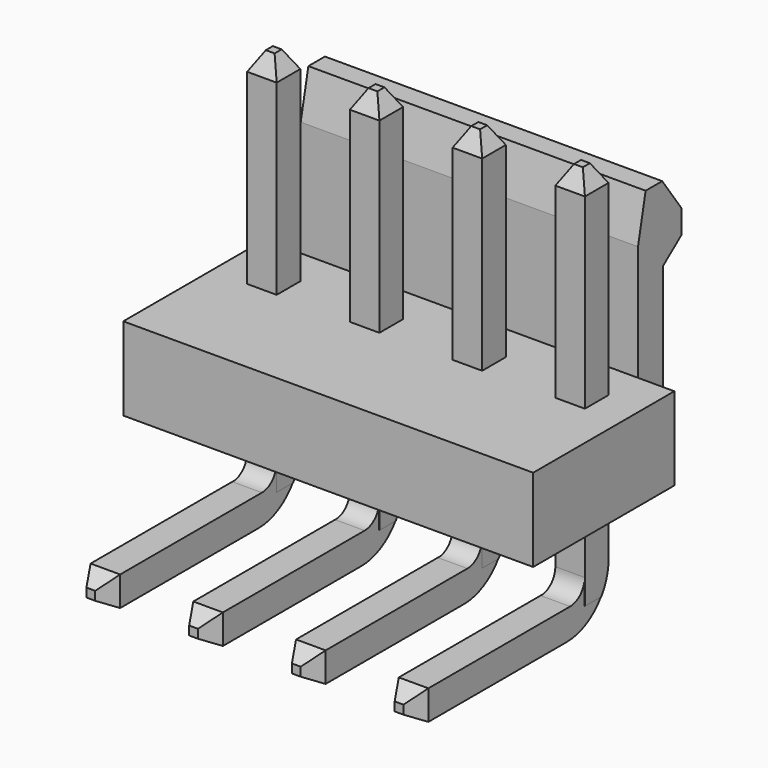
from build123d import *

# Parameters (mm, degrees)
F0_W          = 6.8
F0_H          = 3.2
F1_DEPTH      = 7.9
F1_DEPTH_BACK = 7.9
F2_DEPTH      = 6.5
F2_DEPTH_BACK = 6.5
F3_W          = 1.14
F3_H          = 1.14
F4_DEPTH      = 11.1
F4_DEPTH_BACK = 3.5
F5_C1_SIZE2   = 0.4
F5_C1_SIZE    = 0.7
F5_C2_SIZE2   = 0.7
F5_C2_SIZE    = 0.4
F5_C3_SIZE2   = 0.7
F5_C3_SIZE    = 0.4
F5_C4_SIZE2   = 0.7
F5_C4_SIZE    = 0.4
F5_2_C1_SIZE2 = 0.4
F5_2_C1_SIZE  = 0.7
F5_2_C2_SIZE2 = 0.7
F5_2_C2_SIZE  = 0.4
F5_2_C3_SIZE2 = 0.7
F5_2_C3_SIZE  = 0.4
F5_2_C4_SIZE2 = 0.7
F5_2_C4_SIZE  = 0.4
F5_3_C1_SIZE2 = 0.4
F5_3_C1_SIZE  = 0.7
F5_3_C2_SIZE2 = 0.7
F5_3_C2_SIZE  = 0.4
F5_3_C3_SIZE2 = 0.7
F5_3_C3_SIZE  = 0.4
F5_3_C4_SIZE2 = 0.7
F5_3_C4_SIZE  = 0.4
F5_4_C1_SIZE2 = 0.4
F5_4_C1_SIZE  = 0.7
F5_4_C2_SIZE2 = 0.7
F5_4_C2_SIZE  = 0.4
F5_4_C3_SIZE2 = 0.7
F5_4_C3_SIZE  = 0.4
F5_4_C4_SIZE2 = 0.7
F5_4_C4_SIZE  = 0.4
F6_W          = 1.14
F6_H          = 1.14
F7_DEPTH      = 8.8
F7_DEPTH_BACK = 0.57
F8_R          = 0.7
F8_2_R        = 0.7
F8_3_R        = 0.7
F8_4_R        = 0.7
F9_T1_DEPTH   = 11.14
F9_2_T1_DEPTH = 11.14
F9_3_T1_DEPTH = 11.14
F9_4_T1_DEPTH = 11.14
F10_SIZE2     = 0.7
F10_SIZE      = 0.4
F10_2_SIZE2   = 0.7
F10_2_SIZE    = 0.4
F10_3_SIZE2   = 0.7
F10_3_SIZE    = 0.4
F10_4_SIZE2   = 0.7
F10_4_SIZE    = 0.4


# Not quite as in the source:
# - a fillet or chamfer that OpenCascade refuses, or shapes differently, is made with other operations: its cross-section is extruded or revolved along the edge and cut away or added


with BuildPart() as f1:
    # F0 (on Right) → F1 (new body, two sides)
    with BuildSketch(Plane.YZ) as f1_sk:
        with Locations((-1.4, 1.6)):
            Rectangle(F0_W, F0_H)
    extrude(amount=F1_DEPTH)
    extrude(f1_sk.sketch, amount=-F1_DEPTH_BACK)

    # F0 (on Right) → F2 (join, two sides)
    with BuildSketch(Plane.YZ) as f2_sk:
        Polygon((2, 3.2), (2, 0), (3.2, 0), (3.2, 6.5), (4.1, 7.2), (4.1, 8.1), (3.1672620947, 9.4), (2.3672620947, 9.4), (2, 7.65), align=None)
    extrude(amount=F2_DEPTH)
    extrude(f2_sk.sketch, amount=-F2_DEPTH_BACK)


with BuildPart() as f4:
    # F3 (on Top) → F4 (new body, two sides)
    with BuildSketch(Plane.XY) as f4_sk:
        with Locations((-5.94, 0)):
            Rectangle(F3_W, F3_H)
    extrude(amount=F4_DEPTH)
    extrude(f4_sk.sketch, amount=-F4_DEPTH_BACK)

    # F5: chamfer of 0.7 x 0.4 on 4 edges, made by hand

    # F5_c1
    f5_c1_edges = [f4.edges().sort_by_distance(p)[0] for p in [
        (-5.94, -0.57, 11.1),
    ]]
    f5_c1_side = f4.faces().sort_by_distance((-5.94, -0.57, 11.092))[0]
    chamfer(f5_c1_edges, length=F5_C1_SIZE, length2=F5_C1_SIZE2, reference=f5_c1_side)

    # F5_c2
    f5_c2_edges = [f4.edges().sort_by_distance(p)[0] for p in [
        (-5.94, 0.57, 11.1),
    ]]
    f5_c2_side = f4.faces().sort_by_distance((-5.94, 0.562, 11.1))[0]
    chamfer(f5_c2_edges, length=F5_C2_SIZE, length2=F5_C2_SIZE2, reference=f5_c2_side)

    # F5_c3
    f5_c3_edges = [f4.edges().sort_by_distance(p)[0] for p in [
        (-5.37, 0, 11.1),
    ]]
    f5_c3_side = f4.faces().sort_by_distance((-5.378, 0, 11.1))[0]
    chamfer(f5_c3_edges, length=F5_C3_SIZE, length2=F5_C3_SIZE2, reference=f5_c3_side)

    # F5_c4
    f5_c4_edges = [f4.edges().sort_by_distance(p)[0] for p in [
        (-6.51, 0, 11.1),
    ]]
    f5_c4_side = f4.faces().sort_by_distance((-6.502, 0, 11.1))[0]
    chamfer(f5_c4_edges, length=F5_C4_SIZE, length2=F5_C4_SIZE2, reference=f5_c4_side)

    # F6 (on Front) → F7, piece 4 (join, two sides)
    with BuildSketch(Plane.XZ) as f7_4_sk:
        with Locations((-5.95, -3.8)):
            Rectangle(F6_W, F6_H)
    extrude(amount=F7_DEPTH)
    extrude(f7_4_sk.sketch, amount=-F7_DEPTH_BACK)

    # F8
    f8_edges = [f4.edges().sort_by_distance(p)[0] for p in [
        (-5.945, -0.57, -3.23),
    ]]
    fillet(f8_edges, radius=F8_R)

    # F9: fillet of radius 2 on 1 edges, made by hand

    # F9_s2 → F9_t1 (cut)
    with BuildSketch(Plane.YZ.offset(-11.52)):
        with BuildLine():
            ThreePointArc((0.57, -2.37), (-0.0157864376, -3.7842135624), (-1.43, -4.37))
            Line((-1.43, -4.37), (0.57, -4.37))
            Line((0.57, -4.37), (0.57, -2.37))
        make_face()
    extrude(amount=F9_T1_DEPTH, mode=Mode.SUBTRACT)

    # F10
    f10_edges = [f4.edges().sort_by_distance(p)[0] for p in [
        (-5.38, -8.8, -3.8),
        (-5.95, -8.8, -3.23),
        (-6.52, -8.8, -3.8),
        (-5.95, -8.8, -4.37),
    ]]
    f10_side = f4.faces().sort_by_distance((-5.95, -8.8, -3.8))[0]
    chamfer(f10_edges, length=F10_SIZE, length2=F10_SIZE2, reference=f10_side)


with BuildPart() as f4b:
    # F3 (on Top) → F4, piece 2 (new body, two sides)
    with BuildSketch(Plane.XY) as f4_2_sk:
        with Locations((-1.98, 0)):
            Rectangle(F3_W, F3_H)
    extrude(amount=F4_DEPTH)
    extrude(f4_2_sk.sketch, amount=-F4_DEPTH_BACK)

    # F5#2: chamfer of 0.7 x 0.4 on 4 edges, made by hand

    # F5_2_c1
    f5_2_c1_edges = [f4b.edges().sort_by_distance(p)[0] for p in [
        (-2.55, 0, 11.1),
    ]]
    f5_2_c1_side = f4b.faces().sort_by_distance((-2.55, 0, 11.092))[0]
    chamfer(f5_2_c1_edges, length=F5_2_C1_SIZE, length2=F5_2_C1_SIZE2, reference=f5_2_c1_side)

    # F5_2_c2
    f5_2_c2_edges = [f4b.edges().sort_by_distance(p)[0] for p in [
        (-1.41, 0, 11.1),
    ]]
    f5_2_c2_side = f4b.faces().sort_by_distance((-1.418, 0, 11.1))[0]
    chamfer(f5_2_c2_edges, length=F5_2_C2_SIZE, length2=F5_2_C2_SIZE2, reference=f5_2_c2_side)

    # F5_2_c3
    f5_2_c3_edges = [f4b.edges().sort_by_distance(p)[0] for p in [
        (-1.98, -0.57, 11.1),
    ]]
    f5_2_c3_side = f4b.faces().sort_by_distance((-1.98, -0.562, 11.1))[0]
    chamfer(f5_2_c3_edges, length=F5_2_C3_SIZE, length2=F5_2_C3_SIZE2, reference=f5_2_c3_side)

    # F5_2_c4
    f5_2_c4_edges = [f4b.edges().sort_by_distance(p)[0] for p in [
        (-1.98, 0.57, 11.1),
    ]]
    f5_2_c4_side = f4b.faces().sort_by_distance((-1.98, 0.562, 11.1))[0]
    chamfer(f5_2_c4_edges, length=F5_2_C4_SIZE, length2=F5_2_C4_SIZE2, reference=f5_2_c4_side)

    # F6 (on Front) → F7, piece 3 (join, two sides)
    with BuildSketch(Plane.XZ) as f7_3_sk:
        with Locations((-1.99, -3.8)):
            Rectangle(F6_W, F6_H)
    extrude(amount=F7_DEPTH)
    extrude(f7_3_sk.sketch, amount=-F7_DEPTH_BACK)

    # F8#2
    f8_2_edges = [f4b.edges().sort_by_distance(p)[0] for p in [
        (-1.985, -0.57, -3.23),
    ]]
    fillet(f8_2_edges, radius=F8_2_R)

    # F9#2: fillet of radius 2 on 1 edges, made by hand

    # F9_2_s2 → F9_2_t1 (cut)
    with BuildSketch(Plane.YZ.offset(-7.56)):
        with BuildLine():
            ThreePointArc((0.57, -2.37), (-0.0157864376, -3.7842135624), (-1.43, -4.37))
            Line((-1.43, -4.37), (0.57, -4.37))
            Line((0.57, -4.37), (0.57, -2.37))
        make_face()
    extrude(amount=F9_2_T1_DEPTH, mode=Mode.SUBTRACT)

    # F10#2
    f10_2_edges = [f4b.edges().sort_by_distance(p)[0] for p in [
        (-1.42, -8.8, -3.8),
        (-1.99, -8.8, -3.23),
        (-2.56, -8.8, -3.8),
        (-1.99, -8.8, -4.37),
    ]]
    f10_2_side = f4b.faces().sort_by_distance((-1.99, -8.8, -3.8))[0]
    chamfer(f10_2_edges, length=F10_2_SIZE, length2=F10_2_SIZE2, reference=f10_2_side)


with BuildPart() as f4c:
    # F3 (on Top) → F4, piece 3 (new body, two sides)
    with BuildSketch(Plane.XY) as f4_3_sk:
        with Locations((1.98, 0)):
            Rectangle(F3_W, F3_H)
    extrude(amount=F4_DEPTH)
    extrude(f4_3_sk.sketch, amount=-F4_DEPTH_BACK)

    # F5#3: chamfer of 0.7 x 0.4 on 4 edges, made by hand

    # F5_3_c1
    f5_3_c1_edges = [f4c.edges().sort_by_distance(p)[0] for p in [
        (1.41, 0, 11.1),
    ]]
    f5_3_c1_side = f4c.faces().sort_by_distance((1.41, 0, 11.092))[0]
    chamfer(f5_3_c1_edges, length=F5_3_C1_SIZE, length2=F5_3_C1_SIZE2, reference=f5_3_c1_side)

    # F5_3_c2
    f5_3_c2_edges = [f4c.edges().sort_by_distance(p)[0] for p in [
        (2.55, 0, 11.1),
    ]]
    f5_3_c2_side = f4c.faces().sort_by_distance((2.542, 0, 11.1))[0]
    chamfer(f5_3_c2_edges, length=F5_3_C2_SIZE, length2=F5_3_C2_SIZE2, reference=f5_3_c2_side)

    # F5_3_c3
    f5_3_c3_edges = [f4c.edges().sort_by_distance(p)[0] for p in [
        (1.98, -0.57, 11.1),
    ]]
    f5_3_c3_side = f4c.faces().sort_by_distance((1.98, -0.562, 11.1))[0]
    chamfer(f5_3_c3_edges, length=F5_3_C3_SIZE, length2=F5_3_C3_SIZE2, reference=f5_3_c3_side)

    # F5_3_c4
    f5_3_c4_edges = [f4c.edges().sort_by_distance(p)[0] for p in [
        (1.98, 0.57, 11.1),
    ]]
    f5_3_c4_side = f4c.faces().sort_by_distance((1.98, 0.562, 11.1))[0]
    chamfer(f5_3_c4_edges, length=F5_3_C4_SIZE, length2=F5_3_C4_SIZE2, reference=f5_3_c4_side)

    # F6 (on Front) → F7, piece 2 (join, two sides)
    with BuildSketch(Plane.XZ) as f7_2_sk:
        with Locations((1.97, -3.8)):
            Rectangle(F6_W, F6_H)
    extrude(amount=F7_DEPTH)
    extrude(f7_2_sk.sketch, amount=-F7_DEPTH_BACK)

    # F8#3
    f8_3_edges = [f4c.edges().sort_by_distance(p)[0] for p in [
        (1.975, -0.57, -3.23),
    ]]
    fillet(f8_3_edges, radius=F8_3_R)

    # F9#3: fillet of radius 2 on 1 edges, made by hand

    # F9_3_s2 → F9_3_t1 (cut)
    with BuildSketch(Plane.YZ.offset(-3.6)):
        with BuildLine():
            ThreePointArc((0.57, -2.37), (-0.0157864376, -3.7842135624), (-1.43, -4.37))
            Line((-1.43, -4.37), (0.57, -4.37))
            Line((0.57, -4.37), (0.57, -2.37))
        make_face()
    extrude(amount=F9_3_T1_DEPTH, mode=Mode.SUBTRACT)

    # F10#3
    f10_3_edges = [f4c.edges().sort_by_distance(p)[0] for p in [
        (2.54, -8.8, -3.8),
        (1.97, -8.8, -3.23),
        (1.4, -8.8, -3.8),
        (1.97, -8.8, -4.37),
    ]]
    f10_3_side = f4c.faces().sort_by_distance((1.97, -8.8, -3.8))[0]
    chamfer(f10_3_edges, length=F10_3_SIZE, length2=F10_3_SIZE2, reference=f10_3_side)


with BuildPart() as f4d:
    # F3 (on Top) → F4, piece 4 (new body, two sides)
    with BuildSketch(Plane.XY) as f4_4_sk:
        with Locations((5.94, 0)):
            Rectangle(F3_W, F3_H)
    extrude(amount=F4_DEPTH)
    extrude(f4_4_sk.sketch, amount=-F4_DEPTH_BACK)

    # F5#4: chamfer of 0.7 x 0.4 on 4 edges, made by hand

    # F5_4_c1
    f5_4_c1_edges = [f4d.edges().sort_by_distance(p)[0] for p in [
        (5.37, 0, 11.1),
    ]]
    f5_4_c1_side = f4d.faces().sort_by_distance((5.37, 0, 11.092))[0]
    chamfer(f5_4_c1_edges, length=F5_4_C1_SIZE, length2=F5_4_C1_SIZE2, reference=f5_4_c1_side)

    # F5_4_c2
    f5_4_c2_edges = [f4d.edges().sort_by_distance(p)[0] for p in [
        (6.51, 0, 11.1),
    ]]
    f5_4_c2_side = f4d.faces().sort_by_distance((6.502, 0, 11.1))[0]
    chamfer(f5_4_c2_edges, length=F5_4_C2_SIZE, length2=F5_4_C2_SIZE2, reference=f5_4_c2_side)

    # F5_4_c3
    f5_4_c3_edges = [f4d.edges().sort_by_distance(p)[0] for p in [
        (5.94, -0.57, 11.1),
    ]]
    f5_4_c3_side = f4d.faces().sort_by_distance((5.94, -0.562, 11.1))[0]
    chamfer(f5_4_c3_edges, length=F5_4_C3_SIZE, length2=F5_4_C3_SIZE2, reference=f5_4_c3_side)

    # F5_4_c4
    f5_4_c4_edges = [f4d.edges().sort_by_distance(p)[0] for p in [
        (5.94, 0.57, 11.1),
    ]]
    f5_4_c4_side = f4d.faces().sort_by_distance((5.94, 0.562, 11.1))[0]
    chamfer(f5_4_c4_edges, length=F5_4_C4_SIZE, length2=F5_4_C4_SIZE2, reference=f5_4_c4_side)

    # F6 (on Front) → F7 (join, two sides)
    with BuildSketch(Plane.XZ) as f7_sk:
        with Locations((5.93, -3.8)):
            Rectangle(F6_W, F6_H)
    extrude(amount=F7_DEPTH)
    extrude(f7_sk.sketch, amount=-F7_DEPTH_BACK)

    # F8#4
    f8_4_edges = [f4d.edges().sort_by_distance(p)[0] for p in [
        (5.935, -0.57, -3.23),
    ]]
    fillet(f8_4_edges, radius=F8_4_R)

    # F9#4: fillet of radius 2 on 1 edges, made by hand

    # F9_4_s2 → F9_4_t1 (cut)
    with BuildSketch(Plane.YZ.offset(0.36)):
        with BuildLine():
            ThreePointArc((0.57, -2.37), (-0.0157864376, -3.7842135624), (-1.43, -4.37))
            Line((-1.43, -4.37), (0.57, -4.37))
            Line((0.57, -4.37), (0.57, -2.37))
        make_face()
    extrude(amount=F9_4_T1_DEPTH, mode=Mode.SUBTRACT)

    # F10#4
    f10_4_edges = [f4d.edges().sort_by_distance(p)[0] for p in [
        (6.5, -8.8, -3.8),
        (5.93, -8.8, -3.23),
        (5.36, -8.8, -3.8),
        (5.93, -8.8, -4.37),
    ]]
    f10_4_side = f4d.faces().sort_by_distance((5.93, -8.8, -3.8))[0]
    chamfer(f10_4_edges, length=F10_4_SIZE, length2=F10_4_SIZE2, reference=f10_4_side)


solid = Compound([f1.part, f4.part, f4b.part, f4c.part, f4d.part])
